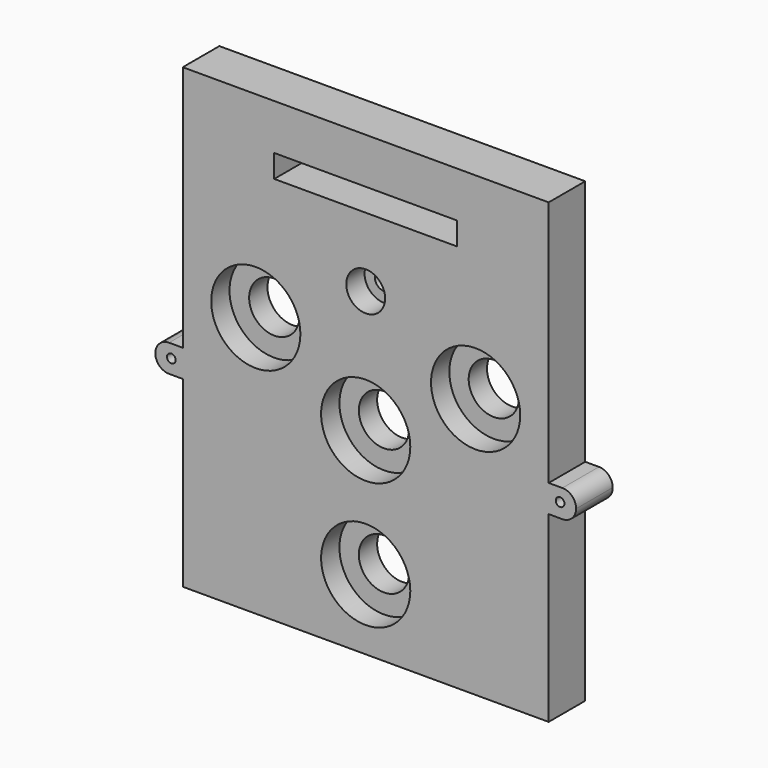
from build123d import *

# Parameters (mm, degrees)
F0_W           = 80
F0_H           = 120
F0_R           = 9.75
F0_R_2         = 4.25
F1_DEPTH       = 5
F2_W           = 80
F2_H           = 120
F2_R           = 5.5
F2_R_2         = 2
F3_DEPTH       = 5
F4_W           = 80
F4_H           = 20
F5_DEPTH       = 10
F6_W           = 6
F6_H           = 6
F6_R           = 0.95
F7_DEPTH       = 10
F8_R           = 2.99999
F11_W          = 40
F11_H          = 5
F12_DEPTH      = 10
F12_DEPTH_BACK = 2
F14_DEPTH      = 0.4
F15_TEXT_SIZE  = 2.2513742958
F16_DEPTH      = 0.4


# Not quite as in the source:
# - a fillet or chamfer is up to 0.001 mm smaller than in the source, because OpenCascade refuses the exact size
# - Text() gives the source's letters only with a copy of the font that has no kerning and outlines rounded to 1/6400 em; it was checked with that copy


with BuildPart() as f1:
    # F0 (on Front) → F1 (new body)
    with BuildSketch(Plane.XZ):
        Rectangle(F0_W, F0_H)
        with Locations((0, -24.624)):
            Circle(F0_R, mode=Mode.SUBTRACT)
        with Locations((-24.032204955, 17.001)):
            Circle(F0_R, mode=Mode.SUBTRACT)
        with Locations((0, 3.126)):
            Circle(F0_R, mode=Mode.SUBTRACT)
        with Locations((0, 29.876)):
            Circle(F0_R_2, mode=Mode.SUBTRACT)
        with Locations((24.032204955, 17.001)):
            Circle(F0_R, mode=Mode.SUBTRACT)
    extrude(amount=F1_DEPTH)

    # F2 (on Front) → F3 (join)
    with BuildSketch(Plane.XZ):
        Rectangle(F2_W, F2_H)
        with Locations((0, -24.6321987361)):
            Circle(F2_R, mode=Mode.SUBTRACT)
        with Locations((-23.9790473133, 17.0061253011)):
            Circle(F2_R, mode=Mode.SUBTRACT)
        with Locations((0, 3.1158635393)):
            Circle(F2_R, mode=Mode.SUBTRACT)
        with Locations((0, 29.8736914992)):
            Circle(F2_R_2, mode=Mode.SUBTRACT)
        with Locations((24.015404284, 16.9426184148)):
            Circle(F2_R, mode=Mode.SUBTRACT)
    extrude(amount=-F3_DEPTH)

    # F4 (on face) → F5 (cut)
    with BuildSketch(Plane.XZ.offset(5)):
        with Locations((0, -50)):
            Rectangle(F4_W, F4_H)
    extrude(amount=-F5_DEPTH, mode=Mode.SUBTRACT)



with BuildPart() as f7:
    # F6 (on face) → F7 (new body)
    with BuildSketch(Plane.XZ.offset(5)):
        with Locations((43, 3)):
            Rectangle(F6_W, F6_H)
        with Locations((42.5, 3.126)):
            Circle(F6_R, mode=Mode.SUBTRACT)
    extrude(amount=-F7_DEPTH)

    # F8 (radius 3 in the source; OpenCascade refuses exactly that, so slightly less here)
    f8_edges = [f7.edges().sort_by_distance(p)[0] for p in [
        (46, 0, 0),
        (46, 0, 6),
    ]]
    fillet(f8_edges, radius=F8_R)


with BuildPart() as f1_1:
    add(f1.part)

    add(f7.part)  # F9 merges F7
    # F9: F7 across plane
    add(f7.part.mirror(Plane.YZ))

    # F11 (on face) → F12 (cut, two sides)
    with BuildSketch(Plane.XZ.offset(5)) as f12_sk:
        with Locations((0, 47.5)):
            Rectangle(F11_W, F11_H)
    extrude(amount=-F12_DEPTH, mode=Mode.SUBTRACT)
    extrude(f12_sk.sketch, amount=F12_DEPTH_BACK, mode=Mode.SUBTRACT)

    # F13 (on face) → F14 (cut)
    with BuildSketch(Plane(origin=(0, 5, 0), x_dir=(-1, 0, 0), z_dir=(0, 1, 0))):
        with BuildLine():
            Line((13.9283005654, -32.2310365663), (14.2649786017, -33.0640835938))
            ThreePointArc((14.2649786017, -33.0640835938), (23.9438238981, -27.5300413453), (31.6548040771, -19.4773117112))
            Line((31.6548040771, -19.4773117112), (32.2561040521, -19.7261891159))
            Line((32.2561040521, -19.7261891159), (32.2561040521, -17.6917891949))
            Line((32.2561040521, -17.6917891949), (30.1847662777, -18.615020439))
            Line((30.1847662777, -18.615020439), (30.9350663638, -18.9391262087))
            ThreePointArc((30.9350663638, -18.9391262087), (23.395494081, -26.8182601396), (13.9283005654, -32.2310365663))
        make_face()
        with BuildLine():
            ThreePointArc((-30.5121443827, -20.4847219412), (-22.8289721503, -27.9778113869), (-13.3787150093, -33.0640835938))
            Line((-13.3787150093, -33.0640835938), (-12.3285112397, -32.2310365663))
            ThreePointArc((-12.3285112397, -32.2310365663), (-22.0316439538, -27.1496647257), (-29.8486845366, -19.4773117112))
            Line((-29.8486845366, -19.4773117112), (-29.0539450943, -18.7158770859))
            Line((-29.0539450943, -18.7158770859), (-31.192438677, -18.7158770859))
            Line((-31.192438677, -18.7158770859), (-31.192438677, -21.3156137615))
            Line((-31.192438677, -21.3156137615), (-30.5121443827, -20.4847219412))
        make_face()
    extrude(amount=-F14_DEPTH, mode=Mode.SUBTRACT)

    # F15 (on face) → F16 (cut)
    with BuildSketch(Plane(origin=(0, 5, 0), x_dir=(-1, 0, 0), z_dir=(0, 1, 0))):
        with Locations(Location((-14.0919930509, -21.979651231), (0, 0, 179.7026547212))):
            Text('HAWSER', F15_TEXT_SIZE, font='Open Sans', font_style=FontStyle.BOLD, text_align=(TextAlign.LEFT, TextAlign.BOTTOM))
        with Locations(Location((-15.8310960664, -18.9087155322), (0, 0, 179.7026547212))):
            Text('(RH)', F15_TEXT_SIZE, font='Open Sans', font_style=FontStyle.BOLD, text_align=(TextAlign.LEFT, TextAlign.BOTTOM))
        with Locations(Location((23.5225135706, -21.9664722681), (0, 0, 179.7026547212))):
            Text('CABLE', F15_TEXT_SIZE, font='Open Sans', font_style=FontStyle.BOLD, text_align=(TextAlign.LEFT, TextAlign.BOTTOM))
        with Locations(Location((22.3684082169, -18.8985725321), (0, 0, 179.7026547212))):
            Text('(LH)', F15_TEXT_SIZE, font='Open Sans', font_style=FontStyle.BOLD, text_align=(TextAlign.LEFT, TextAlign.BOTTOM))
    extrude(amount=-F16_DEPTH, mode=Mode.SUBTRACT)


solid = f1_1.part
